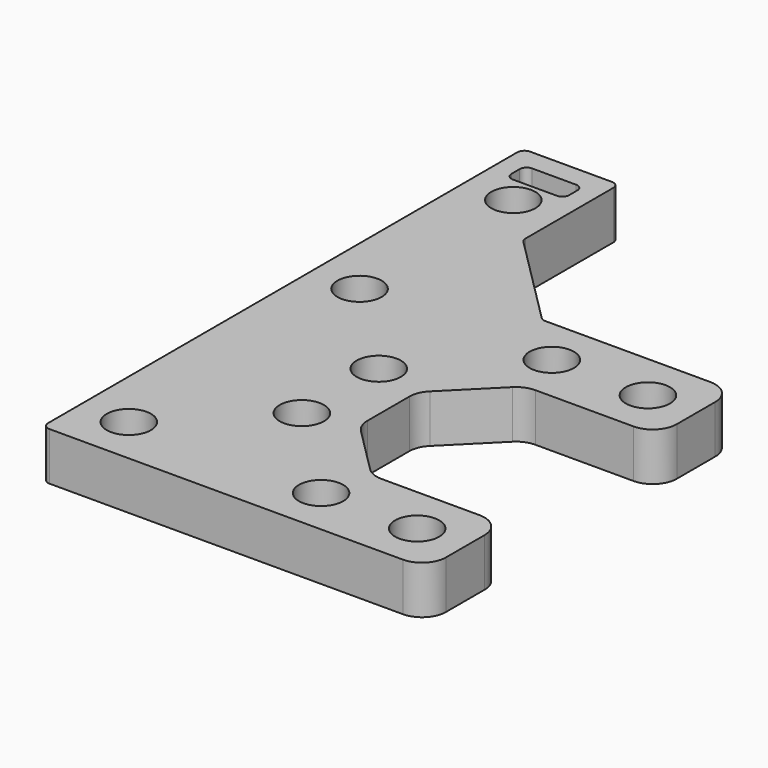
from build123d import *

# Parameters (mm, degrees)
F0_R     = 4.6
F1_DEPTH = 10
F0_R_2   = 2.5
F2_DEPTH = 3


# Not quite as in the source:
# - ends of sketch curves that miss each other by under 0.0002 mm in the source are joined


with BuildPart() as f1:
    # F0 (on Top) → F1 (new body)
    with BuildSketch(Plane.XY):
        with BuildLine():
            ThreePointArc((-40, -61), (-39.5606601718, -62.0606601718), (-38.5, -62.5))
            Line((-38.5, -62.5), (35, -62.5))
            ThreePointArc((35, -62.5), (38.5355339059, -61.0355339059), (40, -57.5))
            Line((40, -57.5), (40, -47.5))
            ThreePointArc((40, -47.5), (38.5355339059, -43.9644660941), (35, -42.5))
            Line((35, -42.5), (14.571067, -42.5))
            ThreePointArc((14.571067, -42.5), (12.6576501648, -42.1193977979), (11.0355335941, -41.0355344059))
            Line((11.0355335941, -41.0355344059), (1.464466, -31.464466))
            ThreePointArc((1.464466, -31.464466), (0.3806023374, -29.8423491618), (0, -27.928932))
            Line((0, -27.928932), (0, -17.071068))
            ThreePointArc((0, -17.071068), (0.3806023374, -15.1576508382), (1.4644660941, -13.5355340941))
            Line((1.4644660941, -13.5355340941), (11.035534, -3.964466))
            ThreePointArc((11.035534, -3.964466), (12.6576501648, -2.8806022021), (14.571067, -2.5))
            Line((14.571067, -2.5), (35, -2.5))
            ThreePointArc((35, -2.5), (38.5355339059, -1.0355339059), (40, 2.5))
            Line((40, 2.5), (40, 12.5))
            ThreePointArc((40, 12.5), (38.5355339059, 16.0355339059), (35, 17.5))
            Line((35, 17.5), (0.62132, 17.5))
            ThreePointArc((0.62132, 17.5), (0.0472948515, 17.6141807012), (-0.4393401718, 17.9393398282))
            Line((-0.4393401718, 17.9393398282), (-19.560661, 37.06066))
            ThreePointArc((-19.560661, 37.06066), (-19.8858192988, 37.5472958515), (-20, 38.121321))
            Line((-20, 38.121321), (-20, 61))
            ThreePointArc((-20, 61), (-20.4393398282, 62.0606601718), (-21.5, 62.5))
            Line((-21.5, 62.5), (-38.5, 62.5))
            ThreePointArc((-38.5, 62.5), (-39.5606601718, 62.0606601718), (-40, 61))
            Line((-40, 61), (-40, -61))
        make_face()
        with Locations((-30, -52.5)):
            Circle(F0_R, mode=Mode.SUBTRACT)
        with Locations((-10, -32.5)):
            Circle(F0_R, mode=Mode.SUBTRACT)
        with Locations((-10, -12.5)):
            Circle(F0_R, mode=Mode.SUBTRACT)
        with Locations((10, -52.5)):
            Circle(F0_R, mode=Mode.SUBTRACT)
        with Locations((30, -52.5)):
            Circle(F0_R, mode=Mode.SUBTRACT)
        with Locations((-30, 7.5)):
            Circle(F0_R, mode=Mode.SUBTRACT)
        with Locations((-30, 47.5)):
            Circle(F0_R, mode=Mode.SUBTRACT)
        with BuildLine():
            Line((-36, 54.53), (-36, 56.65))
            ThreePointArc((-36, 56.65), (-35.5782337649, 57.6682337649), (-34.56, 58.09))
            Line((-34.56, 58.09), (-25.44, 58.09))
            ThreePointArc((-25.44, 58.09), (-24.4217662351, 57.6682337649), (-24, 56.65))
            Line((-24, 56.65), (-24, 54.53))
            ThreePointArc((-24, 54.53), (-24.4217662351, 53.5117662351), (-25.44, 53.09))
            Line((-25.44, 53.09), (-34.56, 53.09))
            ThreePointArc((-34.56, 53.09), (-35.5782337649, 53.5117662351), (-36, 54.53))
        make_face(mode=Mode.SUBTRACT)
        with Locations((10, 7.5)):
            Circle(F0_R, mode=Mode.SUBTRACT)
        with Locations((30, 7.5)):
            Circle(F0_R, mode=Mode.SUBTRACT)
    extrude(amount=F1_DEPTH)

    # F0 (on Top) → F2 (join)
    with BuildSketch(Plane.XY):
        with Locations((-30, 47.5)):
            Circle(F0_R)
        with Locations((-30, 47.5)):
            Circle(F0_R_2, mode=Mode.SUBTRACT)
        with Locations((-30, 7.5)):
            Circle(F0_R)
        with Locations((-30, 7.5)):
            Circle(F0_R_2, mode=Mode.SUBTRACT)
        with Locations((-30, -52.5)):
            Circle(F0_R)
        with Locations((-30, -52.5)):
            Circle(F0_R_2, mode=Mode.SUBTRACT)
        with Locations((-10, -32.5)):
            Circle(F0_R)
        with Locations((-10, -32.5)):
            Circle(F0_R_2, mode=Mode.SUBTRACT)
        with Locations((10, -52.5)):
            Circle(F0_R)
        with Locations((10, -52.5)):
            Circle(F0_R_2, mode=Mode.SUBTRACT)
        with Locations((30, -52.5)):
            Circle(F0_R)
        with Locations((30, -52.5)):
            Circle(F0_R_2, mode=Mode.SUBTRACT)
        with Locations((-10, -12.5)):
            Circle(F0_R)
        with Locations((-10, -12.5)):
            Circle(F0_R_2, mode=Mode.SUBTRACT)
        with Locations((10, 7.5)):
            Circle(F0_R)
        with Locations((10, 7.5)):
            Circle(F0_R_2, mode=Mode.SUBTRACT)
        with Locations((30, 7.5)):
            Circle(F0_R)
        with Locations((30, 7.5)):
            Circle(F0_R_2, mode=Mode.SUBTRACT)
    extrude(amount=F2_DEPTH)


solid = f1.part
